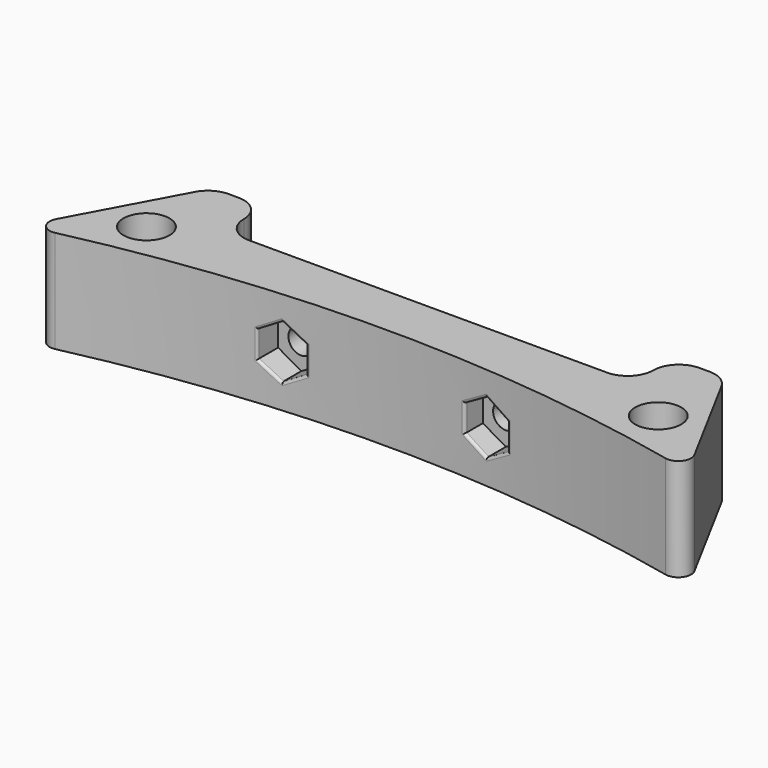
from build123d import *

# Parameters (mm, degrees)
F0_R     = 4.5
F1_DEPTH = 20
F2_R     = 4.99999
F3_R     = 2.5
F4_R     = 2.5
F5_DEPTH = 25
F8_DEPTH = 6
F9_R     = 0.5


# Not quite as in the source:
# - a fillet or chamfer is up to 0.001 mm smaller than in the source, because OpenCascade refuses the exact size
# - a feature names something its author has since deleted; it is built from what else it names


with BuildPart() as f1:
    # F0 (on Top) → F1 (new body)
    with BuildSketch(Plane.XY):
        with BuildLine():
            Line((40, 0), (-40, 0))
            Line((-40, 0), (-40, 10))
            Line((-40, 10), (-50, 10))
            Line((-50, 10), (-65, -17.7922156823))
            ThreePointArc((-65, -17.7922156823), (0, -10), (65, -17.7922156823))
            Line((65, -17.7922156823), (50, 10))
            Line((50, 10), (40, 10))
            Line((40, 10), (40, 0))
        make_face()
        with Locations((-50, -6.2922156823)):
            Circle(F0_R, mode=Mode.SUBTRACT)
        with Locations((50, -6.2922156823)):
            Circle(F0_R, mode=Mode.SUBTRACT)
    extrude(amount=F1_DEPTH)

    # F2 (radius 5 in the source; OpenCascade refuses exactly that, so slightly less here)
    f2_edges = [f1.edges().sort_by_distance(p)[0] for p in [
        (-40, 10, 10),
        (-40, 0, 10),
        (40, 10, 10),
        (40, 0, 10),
        (-50, 10, 10),
        (50, 10, 10),
    ]]
    fillet(f2_edges, radius=F2_R)

    # F3
    f3_edges = [f1.edges().sort_by_distance(p)[0] for p in [
        (-65, -17.792216, 10),
        (65, -17.792216, 10),
    ]]
    fillet(f3_edges, radius=F3_R)

    # F4 (on face) → F5 (cut)
    with BuildSketch(Plane(origin=(0, 0, 0), x_dir=(-1, 0, 0), z_dir=(0, 1, 0))):
        with Locations((-19.9995623863, 10.1323040371)):
            Circle(F4_R)
        with Locations((20, 10)):
            Circle(F4_R)
    extrude(amount=-F5_DEPTH, mode=Mode.SUBTRACT)

    # F7 (on offset) → F8 (cut)
    with BuildSketch(Plane.XZ.offset(12)):
        Polygon((-15.5, 7.4019237886), (-15.5, 12.5980762114), (-20, 15.1961524227), (-24.5, 12.5980762114), (-24.5, 7.4019237886), (-20, 4.8038475773), align=None)
        Polygon((15.5, 12.5980762114), (15.5, 7.4019237886), (20, 4.8038475773), (24.5, 7.4019237886), (24.5, 12.5980762114), (20, 15.1961524227), align=None)
    extrude(amount=-F8_DEPTH, mode=Mode.SUBTRACT)

    # F9
    f9_edges = [f1.edges().sort_by_distance(p)[0] for p in [
        (-22.250563, -10.901637, 13.896789),
        (-24.5, -11.093538, 10),
        (-22.250563, -10.901637, 6.103211),
        (-17.750448, -10.573468, 6.102627),
        (-15.5, -10.437166, 10),
        (-17.750448, -10.573468, 13.897373),
        (17.750448, -10.573468, 13.897373),
        (15.5, -10.437166, 10),
        (17.750448, -10.573468, 6.102627),
        (22.250563, -10.901637, 6.103211),
        (24.5, -11.093538, 10),
        (22.250563, -10.901637, 13.896789),
    ]]
    fillet(f9_edges, radius=F9_R)


solid = f1.part
